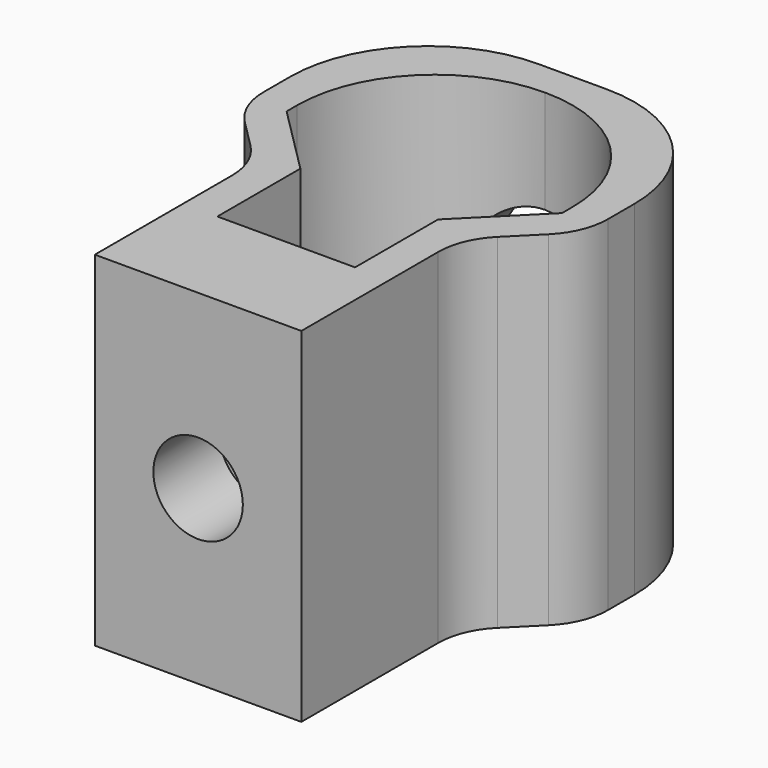
from build123d import *

# Parameters (mm, degrees)
F1_DEPTH    = 25
F2_R        = 5
F3_R        = 3.25
F4_DEPTH    = 6
F5_R        = 1.85
F6_DEPTH    = 2
F7_R        = 5
F8_DEPTH    = 8.9
F9_T1_DEPTH = 75


# Not quite as in the source:
# - a fillet or chamfer that OpenCascade refuses, or shapes differently, is made with other operations: its cross-section is extruded or revolved along the edge and cut away or added


with BuildPart() as f1:
    # F0 (on Top) → F1 (new body)
    with BuildSketch(Plane.XY):
        Polygon((-7.5, 0), (0, 0), (7.5, 0), (7.5, 14.5), (12.5, 19.5), (12.5, 34), (0, 34), (-12.5, 34), (-12.5, 19.5), (-7.5, 14.5), align=None)
        with BuildLine():
            Line((-10, 20.5355339059), (-10, 21.5))
            ThreePointArc((-10, 21.5), (-7.0710678119, 28.5710678119), (0, 31.5))
            ThreePointArc((0, 31.5), (7.0710678119, 28.5710678119), (10, 21.5))
            Line((10, 21.5), (10, 20.5355339059))
            Line((10, 20.5355339059), (5, 15.5355339059))
            Line((5, 15.5355339059), (5, 8))
            Line((5, 8), (-5, 8))
            Line((-5, 8), (-5, 15.5355339059))
            Line((-5, 15.5355339059), (-10, 20.5355339059))
        make_face(mode=Mode.SUBTRACT)
    extrude(amount=F1_DEPTH)

    # F2
    f2_edges = [f1.edges().sort_by_distance(p)[0] for p in [
        (-12.5, 19.5, 12.5),
        (-7.5, 14.5, 12.5),
        (12.5, 19.5, 12.5),
        (7.5, 14.5, 12.5),
    ]]
    fillet(f2_edges, radius=F2_R)

    # F3 (on face) → F4 (cut)
    with BuildSketch(Plane.XZ):
        with Locations((0, 12.5)):
            Circle(F3_R)
    extrude(amount=-F4_DEPTH, mode=Mode.SUBTRACT)

    # F5 (on face) → F6 (cut)
    with BuildSketch(Plane(origin=(0, 8, 0), x_dir=(-1, 0, 0), z_dir=(0, 1, 0))):
        with Locations((0, 12.5)):
            Circle(F5_R)
    extrude(amount=-F6_DEPTH, mode=Mode.SUBTRACT)

    # F7 (on face) → F8 (cut)
    with BuildSketch(Plane(origin=(0, 34, 0), x_dir=(-1, 0, 0), z_dir=(0, 1, 0))):
        with Locations((0, 12.5)):
            Circle(F7_R)
    extrude(amount=-F8_DEPTH, mode=Mode.SUBTRACT)

    # F9: fillet of radius 10 on 2 edges, made by hand

    # F9_s2 → F9_t1 (cut)
    with BuildSketch(Plane.XY.offset(-25)):
        with BuildLine():
            ThreePointArc((-2.5, 34), (-9.5710678119, 31.0710678119), (-12.5, 24))
            Line((-12.5, 24), (-12.5, 34))
            Line((-12.5, 34), (-2.5, 34))
        make_face()
        with BuildLine():
            ThreePointArc((12.5, 24), (9.5710678119, 31.0710678119), (2.5, 34))
            Line((2.5, 34), (12.5, 34))
            Line((12.5, 34), (12.5, 24))
        make_face()
    extrude(amount=F9_T1_DEPTH, mode=Mode.SUBTRACT)


solid = f1.part
